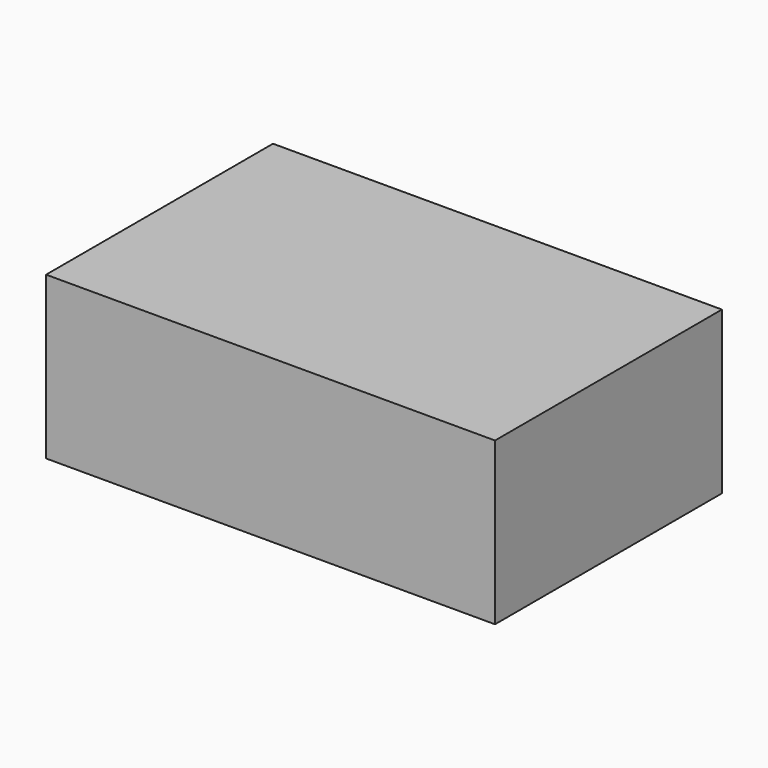
from build123d import *

# Parameters (mm, degrees)
F2_W     = 39.5727823488
F2_H     = 14.2639167607
F3_DEPTH = 25


# Not quite as in the source:
# - the program builds the solid bodies; features that only make, move or delete a surface that nothing else refers to are left out


with BuildPart() as f3:
    # F2 (on Front) → F3 (new body)
    with BuildSketch(Plane.XZ):
        with Locations((-15.3524952475, 68.9210351557)):
            Rectangle(F2_W, F2_H)
    extrude(amount=F3_DEPTH)


solid = f3.part
